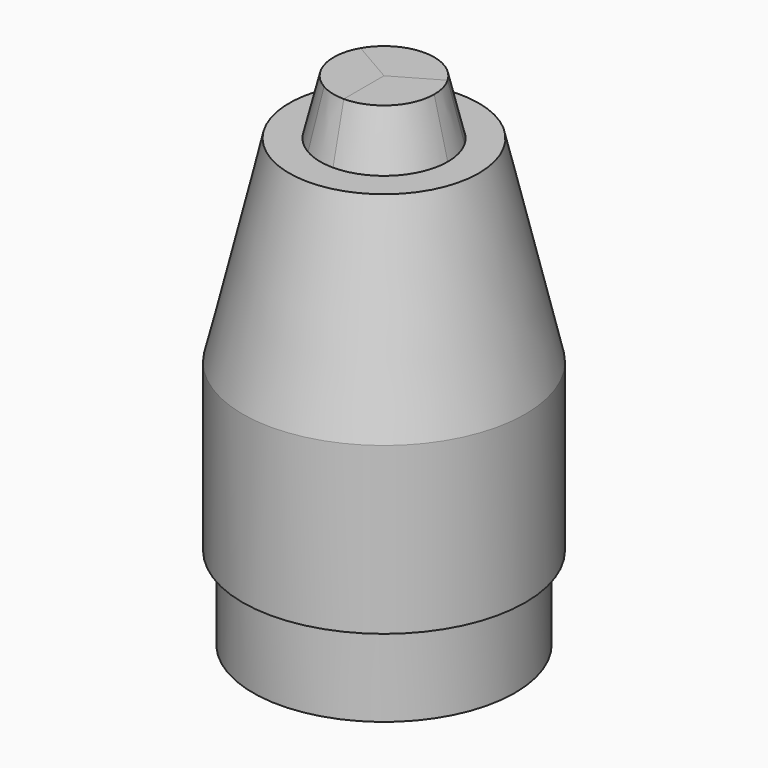
from build123d import *

# Parameters (mm, degrees)
F9_COUNT = 3


with BuildPart() as f1:
    # F0 (on Front) → F1 (revolve)
    with BuildSketch(Plane.XZ):
        Polygon((9.15, 43), (6.15, 43), (11.8165539513, 18.9981087098), (6.1420009622, 19), (6.1356683906, 0), (12.6356683906, 0), (12.6356683906, 8), (13.6356683906, 8), (13.6356683906, 24), align=None)
    revolve(axis=Axis((0, 0, 18.9958373085), (0, 0, -1)))


with BuildPart() as f8:
    # F4 (on offset) → F8 section 0
    with BuildSketch(Plane.XY.offset(30.7)):
        with BuildLine():
            ThreePointArc((0, -9.15), (6.4700270479, -6.4700270479), (9.15, 0))
            ThreePointArc((9.15, 0), (8.8382213105, 2.3681942627), (7.9241324446, 4.575))
            Line((7.9241324446, 4.575), (5.3260562333, 3.075))
            Line((5.3260562333, 3.075), (0, 0))
            Line((0, 0), (0, -9.15))
        make_face()
    # F7 (on offset) → F8 section 1
    with BuildSketch(Plane.XY.offset(48.3)):
        with BuildLine():
            ThreePointArc((0, -4.849200137), (3.4289023002, -3.4289023002), (4.849200137, 0))
            ThreePointArc((4.849200137, 0), (4.6839676491, 1.255065349), (4.1995305066, 2.4246000685))
            Line((4.1995305066, 2.4246000685), (0, 0))
            Line((0, 0), (0, -4.849200137))
        make_face()
    loft()


with BuildPart() as f9_1:
    # F9: instance of F8
    add(f8.part.rotate(Axis((0, 0, 43), (0, 0, -1)), 1 * 360 / F9_COUNT))


with BuildPart() as f9_2:
    # F9: instance of F8
    add(f8.part.rotate(Axis((0, 0, 43), (0, 0, -1)), 2 * 360 / F9_COUNT))


solid = Compound([f1.part, f8.part, f9_1.part, f9_2.part])
